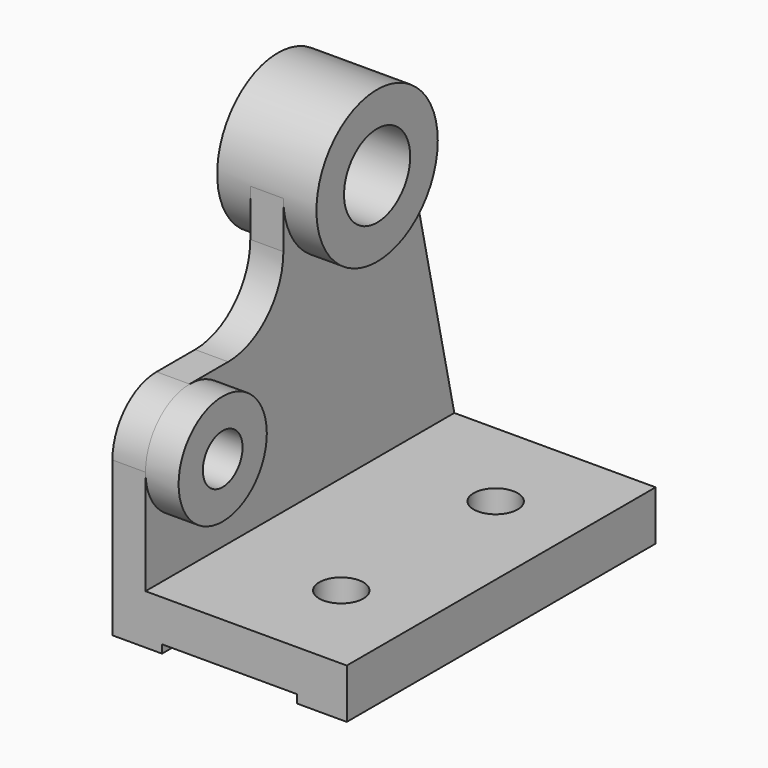
from build123d import *

# Parameters (mm, degrees)
F0_W      = 85
F0_H      = 140
F0_R      = 8
F1_DEPTH  = 18
F2_W      = 49
F2_H      = 3
F3_DEPTH  = 140.001
F4_W      = 12
F4_H      = 140
F5_DEPTH  = 100
F6_R      = 9
F7_DEPTH  = 12
F9_R      = 27.5
F9_R_2    = 15
F10_DEPTH = 18
F11_DEPTH = 25
F12_DEPTH = 25
F13_R     = 25
F14_DEPTH = 25


with BuildPart() as f1:
    # F0 (on Top) → F1 (new body)
    with BuildSketch(Plane.XY):
        with Locations((42.5, 0)):
            Rectangle(F0_W, F0_H)
        with Locations((55, -35)):
            Circle(F0_R, mode=Mode.SUBTRACT)
        with Locations((55, 35)):
            Circle(F0_R, mode=Mode.SUBTRACT)
    extrude(amount=F1_DEPTH)

    # F2 (on face) → F3 (cut, through all)
    with BuildSketch(Plane.XZ.offset(70)):
        with Locations((42.5, 1.5)):
            Rectangle(F2_W, F2_H)
    extrude(amount=-F3_DEPTH, mode=Mode.SUBTRACT)

    # F4 (on face) → F5 (join)
    with BuildSketch(Plane.XY.offset(18)):
        with Locations((6, 0)):
            Rectangle(F4_W, F4_H)
    extrude(amount=F5_DEPTH)

    # F6 (on face) → F7 (join)
    with BuildSketch(Plane.YZ.offset(12)):
        with BuildLine():
            ThreePointArc((-30, 56), (-35.8578643763, 70.1421356237), (-50, 76))
            ThreePointArc((-50, 76), (-64.1421356237, 70.1421356237), (-70, 56))
            ThreePointArc((-70, 56), (-50, 36), (-30, 56))
        make_face()
        with Locations((-50, 56)):
            Circle(F6_R, mode=Mode.SUBTRACT)
    extrude(amount=F7_DEPTH)

    # F9 (on offset) → F10 (join, symmetric)
    with BuildSketch(Plane.YZ.offset(6)):
        with Locations((20, 118)):
            Circle(F9_R)
        with Locations((20, 118)):
            Circle(F9_R_2, mode=Mode.SUBTRACT)
    extrude(amount=F10_DEPTH, both=True)

    # F6 (on face) → F11 (cut)
    with BuildSketch(Plane.YZ.offset(12)):
        with Locations((-50, 56)):
            Circle(F6_R)
        with BuildLine():
            ThreePointArc((5, 118), (20, 103), (35, 118))
            Line((35, 118), (20, 118))
            Line((20, 118), (5, 118))
        make_face()
    extrude(amount=-F11_DEPTH, mode=Mode.SUBTRACT)

    # F6 (on face) → F12 (cut)
    with BuildSketch(Plane.YZ.offset(12)):
        with BuildLine():
            Line((-7.5, 76), (-7.5, 118))
            Line((-7.5, 118), (-70, 118))
            Line((-70, 118), (-70, 56))
            ThreePointArc((-70, 56), (-64.1421356237, 70.1421356237), (-50, 76))
            Line((-50, 76), (-7.5, 76))
        make_face()
        Polygon((70, 118), (47.5, 118), (70, 18), align=None)
    extrude(amount=-F12_DEPTH, mode=Mode.SUBTRACT)

    # F13
    f13_edges = [f1.edges().sort_by_distance(p)[0] for p in [
        (6, -7.5, 76),
    ]]
    fillet(f13_edges, radius=F13_R)

    # F0 (on Top) → F14 (cut)
    with BuildSketch(Plane.XY):
        with Locations((55, -35)):
            Circle(F0_R)
        with Locations((55, 35)):
            Circle(F0_R)
    extrude(amount=-F14_DEPTH, mode=Mode.SUBTRACT)


solid = f1.part
